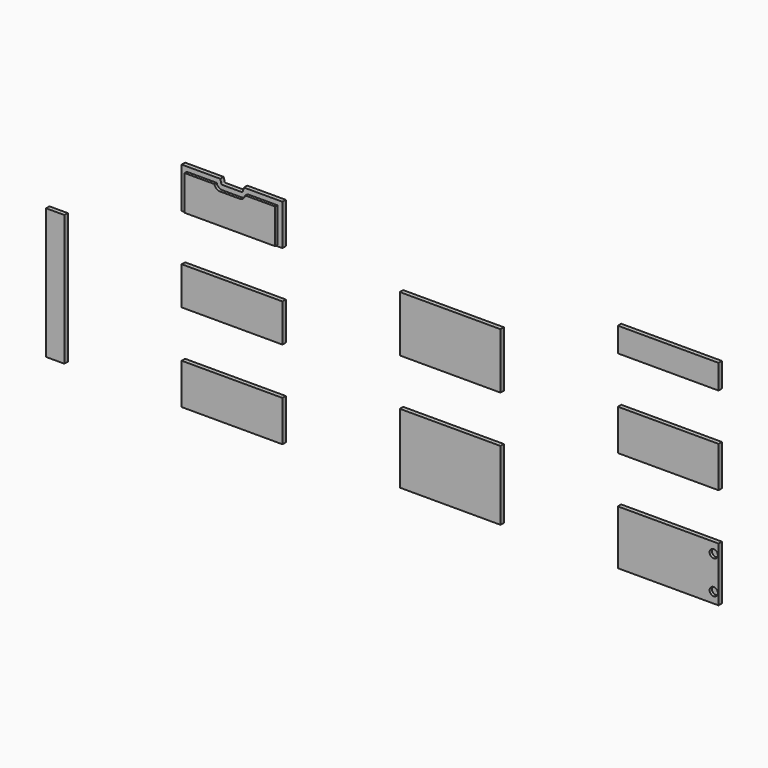
from build123d import *

# Parameters (mm, degrees)
F1_W     = 78
F1_H     = 558
F2_DEPTH = 18
F1_W_2   = 429.33
F1_H_2   = 174
F1_H_3   = 162
F1_H_4   = 238
F1_H_5   = 296
F1_H_6   = 104
F1_H_7   = 232
F3_R     = 17.5
F4_DEPTH = 12
F6_DEPTH = 18
F8_DEPTH = 12


# Not quite as in the source:
# - a feature names something its author has since deleted; it is built from what else it names


with BuildPart() as f2:
    # F1 (on Front) → F2 (new body)
    with BuildSketch(Plane.XZ):
        with Locations((-539, -457)):
            Rectangle(F1_W, F1_H)
    extrude(amount=F2_DEPTH)


with BuildPart() as f2b:
    # F1 (on Front) → F2, piece 2 (new body)
    with BuildSketch(Plane.XZ):
        with Locations((214.665, 87)):
            Rectangle(F1_W_2, F1_H_2)
    extrude(amount=F2_DEPTH)

    # F5 (on face) → F6 (cut)
    with BuildSketch(Plane.XZ.offset(18)):
        with BuildLine():
            ThreePointArc((168.6720058084, 157.7059047745), (170.4578277949, 155.0332332985), (173.5016349399, 154))
            Line((173.5016349399, 154), (214.665, 154))
            Line((214.665, 154), (255.8283650601, 154))
            ThreePointArc((255.8283650601, 154), (258.8721722051, 155.0332332985), (260.6579941916, 157.7059047745))
            Line((260.6579941916, 157.7059047745), (265.0239838486, 174))
            Line((265.0239838486, 174), (164.3060161514, 174))
            Line((164.3060161514, 174), (168.6720058084, 157.7059047745))
        make_face()
    extrude(amount=-F6_DEPTH, mode=Mode.SUBTRACT)


with BuildPart() as f2c:
    # F1 (on Front) → F2, piece 3 (new body)
    with BuildSketch(Plane.XZ):
        with Locations((214.665, -281)):
            Rectangle(F1_W_2, F1_H_3)
    extrude(amount=F2_DEPTH)


with BuildPart() as f2d:
    # F1 (on Front) → F2, piece 4 (new body)
    with BuildSketch(Plane.XZ):
        with Locations((214.665, -649)):
            Rectangle(F1_W_2, F1_H_2)
    extrude(amount=F2_DEPTH)


with BuildPart() as f2e:
    # F1 (on Front) → F2, piece 5 (new body)
    with BuildSketch(Plane.XZ):
        with Locations((1143.995, -121)):
            Rectangle(F1_W_2, F1_H_4)
    extrude(amount=F2_DEPTH)


with BuildPart() as f2f:
    # F1 (on Front) → F2, piece 6 (new body)
    with BuildSketch(Plane.XZ):
        with Locations((1143.995, -588)):
            Rectangle(F1_W_2, F1_H_5)
    extrude(amount=F2_DEPTH)


with BuildPart() as f2g:
    # F1 (on Front) → F2, piece 7 (new body)
    with BuildSketch(Plane.XZ):
        with Locations((2073.325, 122)):
            Rectangle(F1_W_2, F1_H_6)
    extrude(amount=F2_DEPTH)


with BuildPart() as f2h:
    # F1 (on Front) → F2, piece 8 (new body)
    with BuildSketch(Plane.XZ):
        with Locations((2073.325, -217)):
            Rectangle(F1_W_2, F1_H_2)
    extrude(amount=F2_DEPTH)


with BuildPart() as f2i:
    # F1 (on Front) → F2, piece 9 (new body)
    with BuildSketch(Plane.XZ):
        with Locations((2073.325, -620)):
            Rectangle(F1_W_2, F1_H_7)
    extrude(amount=F2_DEPTH)

    # F3 (on face) → F4 (cut)
    with BuildSketch(Plane.XZ.offset(18)):
        with Locations((2267.49, -549)):
            Circle(F3_R)
        with Locations((2267.49, -691)):
            Circle(F3_R)
    extrude(amount=-F4_DEPTH, mode=Mode.SUBTRACT)


with BuildPart() as f8:
    # F7 (on face) → F8 (new body)
    with BuildSketch(Plane.XZ.offset(18)):
        with BuildLine():
            Line((22, 154), (22, 5))
            Line((22, 5), (407.33, 5))
            Line((407.33, 5), (407.33, 154))
            Line((407.33, 154), (280.3705236082, 154))
            Line((280.3705236082, 154), (279.9765107173, 152.5295238724))
            ThreePointArc((279.9765107173, 152.5295238724), (271.0474007853, 139.1661664927), (255.8283650601, 134))
            Line((255.8283650601, 134), (173.5016349399, 134))
            ThreePointArc((173.5016349399, 134), (158.2825992147, 139.1661664927), (149.3534892827, 152.5295238724))
            Line((149.3534892827, 152.5295238724), (148.9594763918, 154))
            Line((148.9594763918, 154), (22, 154))
        make_face()
    extrude(amount=F8_DEPTH)


solid = Compound([f2.part, f2b.part, f2c.part, f2d.part, f2e.part, f2f.part, f2g.part, f2h.part, f2i.part, f8.part])
